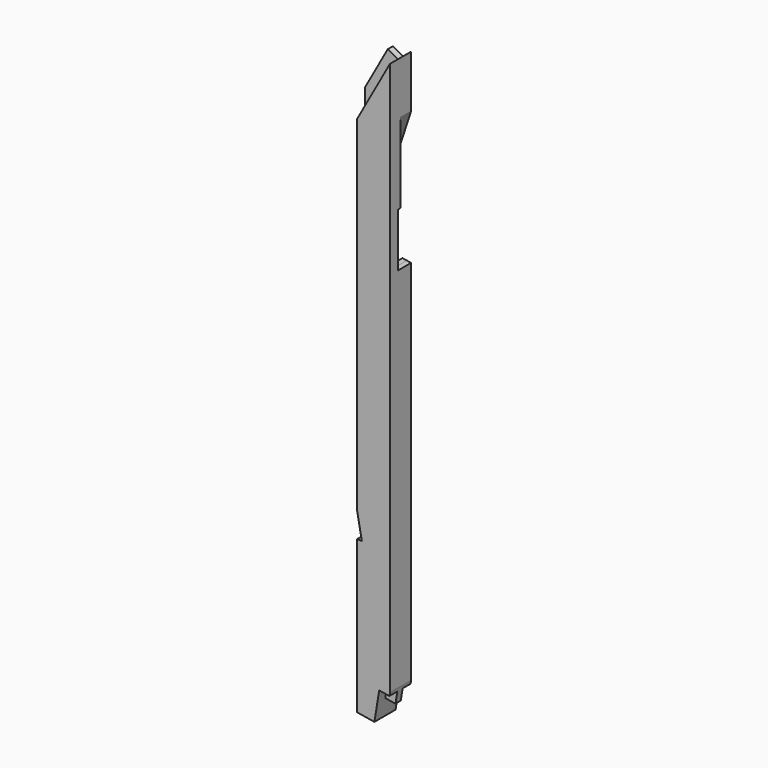
from build123d import *

# Parameters (mm, degrees)
F1_DEPTH = 101.6
F2_DEPTH = 25.4
F4_DEPTH = 127
F5_DEPTH = 101.6
F6_W     = 50.8
F6_H     = 609.6
F7_DEPTH = 114.3


# Not quite as in the source:
# - a feature names something its author has since deleted; it is built from what else it names


with BuildPart() as f1:
    # F0 (on Front) → F1 (new body, symmetric)
    with BuildSketch(Plane.XZ):
        Polygon((48.6763836202, -2036.5928072073), (-127, -2007.7116097401), (-127, -2265.1212), (7.4718955151, -2287.2283796227), (30.1343639729, -2149.3788147942), (44.5559348097, -2061.6563644488), align=None)
        Polygon((122.8795511895, -2074.5327669817), (127, -2049.4692097401), (48.6763836202, -2036.5928072073), (44.5559348097, -2061.6563644488), align=None)
        Polygon((127, -2049.4692097401), (127, -1560.1717829992), (48.6763836202, -2036.5928072073), align=None)
        Polygon((127, 2201.4217376709), (-127, 1744.0764904022), (-127, -892.4533128738), (-88.955976069, -1095.0152873993), (-127, -1095.0152873993), (-127, -2007.7116097401), (48.6763836202, -2036.5928072073), (127, -1560.1717829992), (127, 1433.3240232688), align=None)
    extrude(amount=F1_DEPTH, both=True)

    # F0 (on Front) → F2 (join, symmetric)
    with BuildSketch(Plane.XZ):
        Polygon((108.4579803527, -2162.2552173271), (122.8795511895, -2074.5327669817), (44.5559348097, -2061.6563644488), (30.1343639729, -2149.3788147942), align=None)
        Polygon((49.2815975347, 2244.584915476), (-127, 1927.1772351083), (-127, 1744.0764904022), (127, 2201.4217376709), align=None)
    extrude(amount=F2_DEPTH, both=True)

    # F3 (on face) → F4 (cut)
    with BuildSketch(Plane(origin=(0, 101.6, 0), x_dir=(-1, 0, 0), z_dir=(0, 1, 0))):
        Polygon((-127, 979.0334624678), (-94.0364095159, 778.5250045355), (-60.5988418361, 784.022140662), (-124.8374418386, 979.3889870295), align=None)
        Polygon((-127, 979.0334624678), (-127, 773.1057902599), (-94.0364095159, 778.5250045355), align=None)
        Polygon((-124.8374418386, 979.3889870295), (-60.5988418361, 784.022140662), (127, 814.8633902599), (127, 1020.7910624678), align=None)
        Polygon((64.588744063, 1216.4583241996), (127, 1026.6494750977), (127, 1226.7187346757), align=None)
        Polygon((-127, 985.9659075737), (-127, 979.0334624678), (-124.8374418386, 979.3889870295), align=None)
        Polygon((-127, 985.9659075737), (-124.8374418386, 979.3889870295), (127, 1020.7910624678), (127, 1026.6494750977), (64.588744063, 1216.4583241996), (-127, 1184.9611346757), align=None)
    extrude(amount=-F4_DEPTH, mode=Mode.SUBTRACT)

    # F3 (on face) → F5 (cut)
    with BuildSketch(Plane(origin=(0, 101.6, 0), x_dir=(-1, 0, 0), z_dir=(0, 1, 0))):
        Polygon((-60.5988418361, 784.022140662), (-57.0094351378, 773.1057902599), (127, 773.1057902599), (127, 814.8633902599), align=None)
        Polygon((127, 773.1057902599), (-57.0094351378, 773.1057902599), (127, 213.483646512), align=None)
        Polygon((-127, 1799.129486084), (-127, 1184.9611346757), (64.588744063, 1216.4583241996), align=None)
    extrude(amount=-F5_DEPTH, mode=Mode.SUBTRACT)

    # F6 (on face) → F7 (cut)
    with BuildSketch(Plane(origin=(-127, 0, 0), x_dir=(0, -1, 0), z_dir=(-1, 0, 0))):
        with Locations((0, -1399.8152873993)):
            Rectangle(F6_W, F6_H)
    extrude(amount=-F7_DEPTH, mode=Mode.SUBTRACT)


solid = f1.part
